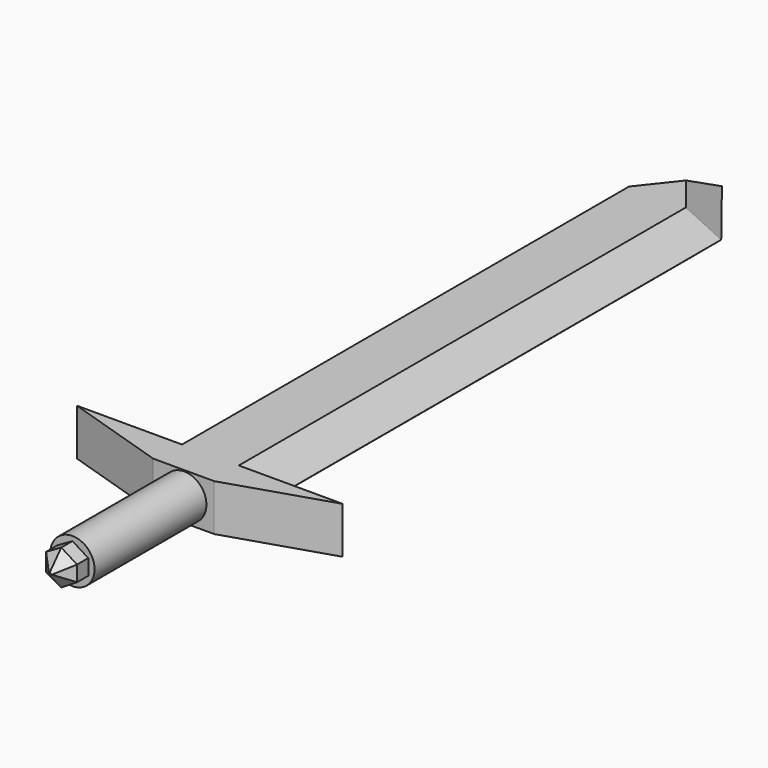
from build123d import *

# Parameters (mm, degrees)
F1_DEPTH = 5
F2_SIZE2 = 5.958758
F2_SIZE  = 4.99999
F4_R     = 4.75
F5_DEPTH = 30
F7_DEPTH = 6
F8_SIZE2 = 3
F8_SIZE  = 3


# Not quite as in the source:
# - a fillet or chamfer is up to 0.001 mm smaller than in the source, because OpenCascade refuses the exact size


with BuildPart() as f1:
    # F0 (on Top) → F1 (new body)
    with BuildSketch(Plane.XY):
        Polygon((-12.0511064306, 53.3692054451), (-12.0511064306, -68.6175450683), (12.0511064306, -68.6175450683), (12.0511064306, 53.3692054451), (0, 68.6175450683), align=None)
        Polygon((12.0511064306, -68.6175450683), (-12.0511064306, -68.6175450683), (-28.6420956254, -68.6175450683), (-6.6773975268, -75.6341889501), (6.4345644787, -75.6341889501), (28.3992625773, -68.6175450683), align=None)
    extrude(amount=F1_DEPTH)

    # F2 (size 5 and 5.958767963 in the source; OpenCascade refuses exactly that, so slightly less here)
    f2_edges = [f1.edges().sort_by_distance(p)[0] for p in [
        (12.051106, -7.62417, 5),
        (6.025553, 60.993375, 5),
        (-6.025553, 60.993375, 5),
        (-12.051106, -7.62417, 5),
    ]]
    chamfer(f2_edges, length=F2_SIZE, length2=F2_SIZE2)

    # F3: F1 across plane


with BuildPart() as f1_1:
    add(f1.part)
    add(f1.part.mirror(Plane.XY))

    # F4 (on face) → F5 (join)
    with BuildSketch(Plane.XZ.offset(75.6341889501)):
        Circle(F4_R)
    extrude(amount=F5_DEPTH)

    # F6 (on face) → F7 (join)
    with BuildSketch(Plane.XZ.offset(105.6341889501)):
        Polygon((3.3913787161, 1.6732233375), (0, 3.7816829499), (-3.2607477523, 1.9153720341), (-3.2607477523, -1.9153720341), (0, -3.7816829499), (3.3913787161, -1.6732233375), align=None)
    extrude(amount=F7_DEPTH)

    # F8
    f8_edges = [f1_1.edges().sort_by_distance(p)[0] for p in [
        (-1.630374, -111.634189, 2.848527),
        (1.695689, -111.634189, 2.727453),
        (-3.260748, -111.634189, 0),
        (-1.630374, -111.634189, -2.848527),
        (1.695689, -111.634189, -2.727453),
        (3.391379, -111.634189, 0),
    ]]
    chamfer(f8_edges, length=F8_SIZE, length2=F8_SIZE2)


solid = f1_1.part
